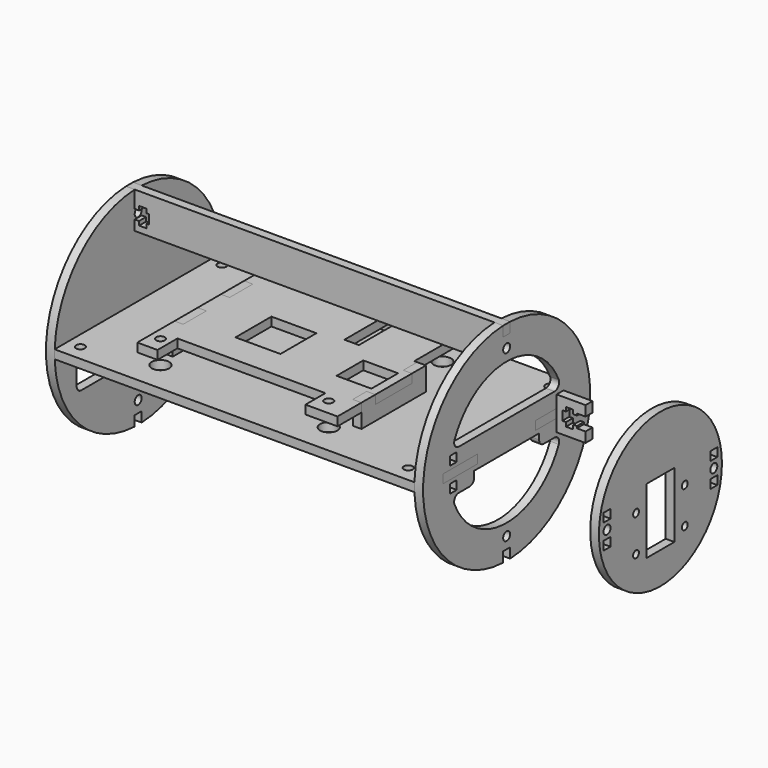
from build123d import *

# Parameters (mm, degrees)
F0_W      = 3
F0_H      = 15
F1_DEPTH  = 3
F3_R      = 1.5
F3_W      = 15.5
F3_H      = 15.5
F3_W_2    = 12
F3_H_2    = 11.5
F4_DEPTH  = 3
F5_W      = 3
F5_H      = 6
F5_W_2    = 10
F5_H_2    = 3
F5_W_3    = 7
F5_H_3    = 10
F6_DEPTH  = 25
F5_R      = 3
F5_R_2    = 1.5
F7_DEPTH  = 25
F9_DEPTH  = 3
F11_DEPTH = 3
F13_DEPTH = 3
F14_R     = 36
F14_W     = 25
F14_H     = 3
F15_DEPTH = 3
F16_R     = 2
F17_R     = 36
F17_W     = 15
F17_H     = 3
F18_DEPTH = 3
F19_R     = 1.5
F19_W     = 3
F19_H     = 7
F20_DEPTH = 130.001
F22_DEPTH = 3
F23_W     = 3
F23_H     = 3
F24_DEPTH = 3
F26_R     = 26.5
F26_W     = 3
F26_H     = 3
F26_R_2   = 1.25
F26_W_2   = 12
F26_H_2   = 22.5
F26_R_3   = 1.5
F27_DEPTH = 3
F28_R     = 1.524
F28_R_2   = 3
F29_DEPTH = 25


with BuildPart() as f1:
    # F0 (on Top) → F1 (new body)
    with BuildSketch(Plane.XY):
        Polygon((62, 36), (-62, 36), (-62, 27.5), (-62, 12.5), (-62, -12.5), (-62, -27.5), (-62, -36), (62, -36), (62, -27.5), (62, -12.5), (62, 12.5), (62, 27.5), align=None)
        with Locations((-63.5, 20)):
            Rectangle(F0_W, F0_H)
        with Locations((63.5, 20)):
            Rectangle(F0_W, F0_H)
        with Locations((-63.5, -20)):
            Rectangle(F0_W, F0_H)
        with Locations((63.5, -20)):
            Rectangle(F0_W, F0_H)
    extrude(amount=F1_DEPTH)


with BuildPart() as f4:
    # F3 (on offset) → F4 (new body)
    with BuildSketch(Plane(origin=(0, 0, 8), x_dir=(1, 0, 0), z_dir=(0, 0, -1))):
        Polygon((-37.5, 31), (-37.5, -31), (5, -31), (5, -5.1), (10, -5.1), (10, -31), (27.5, -31), (27.5, -7.1), (31.5, -7.1), (31.5, 31), (20.45, 31), (20.45, 22.4), (-30.55, 22.4), (-30.55, 31), align=None)
        with Locations((-34, -23.6)):
            Circle(F3_R, mode=Mode.SUBTRACT)
        with Locations((24, -23.6)):
            Circle(F3_R, mode=Mode.SUBTRACT)
        with Locations((-11, 4.4)):
            Rectangle(F3_W, F3_H, mode=Mode.SUBTRACT)
        with Locations((-34, 25.4)):
            Circle(F3_R, mode=Mode.SUBTRACT)
        with Locations((22.5, 6.9)):
            Rectangle(F3_W_2, F3_H_2, mode=Mode.SUBTRACT)
        with Locations((24, 25.4)):
            Circle(F3_R, mode=Mode.SUBTRACT)
    extrude(amount=-F4_DEPTH)


with BuildPart() as f6_tool:
    # F5 (on face) → F6 (new body)
    with BuildSketch(Plane.XY.offset(11)):
        with Locations((30, -17.68)):
            Rectangle(F5_W, F5_H)
        with Locations((30, 4.1)):
            Rectangle(F5_W, F5_H)
        with Locations((0, 29.5)):
            Rectangle(F5_W_2, F5_H_2)
        with Locations((-28, 29.5)):
            Rectangle(F5_W_3, F5_H_2)
        with Locations((-36, 10)):
            Rectangle(F5_W, F5_H_3)
        with Locations((-36, -10)):
            Rectangle(F5_W, F5_H_3)
    extrude(amount=-F6_DEPTH)


with BuildPart() as f1_1:
    add(f1.part)

    # F6: cut by f6_tool
    add(f6_tool.part, mode=Mode.SUBTRACT)

    # F5 (on face) → F7 (cut)
    with BuildSketch(Plane.XY.offset(11)):
        with Locations((24, -25.4)):
            Circle(F5_R)
        with Locations((24, -25.4)):
            Circle(F5_R_2, mode=Mode.SUBTRACT)
        with Locations((-34, -25.4)):
            Circle(F5_R)
        with Locations((-34, -25.4)):
            Circle(F5_R_2, mode=Mode.SUBTRACT)
        with Locations((24, 23.6)):
            Circle(F5_R)
        with Locations((24, 23.6)):
            Circle(F5_R_2, mode=Mode.SUBTRACT)
        with Locations((-34, 23.6)):
            Circle(F5_R)
        with Locations((-34, 23.6)):
            Circle(F5_R_2, mode=Mode.SUBTRACT)
    extrude(amount=-F7_DEPTH, mode=Mode.SUBTRACT)

    # F28 (on face) → F29 (cut)
    with BuildSketch(Plane(origin=(0, 0, 0), x_dir=(1, 0, 0), z_dir=(0, 0, -1))):
        with Locations((55.5, -30.5)):
            Circle(F28_R)
        with Locations((-57.5, -30.5)):
            Circle(F28_R)
        with Locations((-57.5, 30.5)):
            Circle(F28_R)
        with Locations((55.5, 30.5)):
            Circle(F28_R)
        with Locations((-34, 25.4)):
            Circle(F28_R_2)
        with Locations((24, 25.4)):
            Circle(F28_R_2)
        with Locations((-34, -23.6)):
            Circle(F28_R_2)
        with Locations((24, -23.6)):
            Circle(F28_R_2)
    extrude(amount=-F29_DEPTH, mode=Mode.SUBTRACT)


with BuildPart() as f4_1:
    add(f4.part)

    # F6: cut by f6_tool
    add(f6_tool.part, mode=Mode.SUBTRACT)


with BuildPart() as f9:
    # F8 (on face) → F9 (new body)
    with BuildSketch(Plane(origin=(-34.5, 0, 0), x_dir=(0, -1, 0), z_dir=(-1, 0, 0))):
        Polygon((5, 0), (15, 0), (15, 3), (19.5, 3), (19.5, 8), (15, 8), (15, 11), (5, 11), (5, 8), (-5, 8), (-5, 11), (-15, 11), (-15, 8), (-19.5, 8), (-19.5, 3), (-15, 3), (-15, 0), (-5, 0), (-5, 3), (5, 3), align=None)
    extrude(amount=F9_DEPTH)


with BuildPart() as f11:
    # F10 (on face) → F11 (new body)
    with BuildSketch(Plane(origin=(0, 28, 0), x_dir=(-1, 0, 0), z_dir=(0, 1, 0))):
        Polygon((5, 11), (-5, 11), (-5, 0), (5, 0), (5, 3), (24.5, 3), (24.5, 0), (31.5, 0), (31.5, 11), (24.5, 11), (24.5, 8), (5, 8), align=None)
    extrude(amount=F11_DEPTH)


with BuildPart() as f13:
    # F12 (on face) → F13 (new body)
    with BuildSketch(Plane.YZ.offset(28.5)):
        Polygon((7.1, 0), (7.1, 11), (1.1, 11), (1.1, 8), (-14.68, 8), (-14.68, 11), (-20.68, 11), (-20.68, 0), (-14.68, 0), (-14.68, 3), (1.1, 3), (1.1, 0), align=None)
    extrude(amount=F13_DEPTH)


with BuildPart() as f15:
    # F14 (on face) → F15 (new body)
    with BuildSketch(Plane.YZ.offset(62)):
        with Locations((0, 1.5)):
            Circle(F14_R)
        with BuildLine():
            ThreePointArc((-23.4787137637, 8.5), (0, 26), (23.4787137637, 8.5))
            ThreePointArc((23.4787137637, 8.5), (23.6554641744, 7.8772262541), (23.8156986041, 7.25))
            Line((23.8156986041, 7.25), (24.5, 7.25))
            Line((24.5, 7.25), (24.5, 4.25))
            Line((24.5, 4.25), (24.3451740598, 4.25))
            ThreePointArc((24.3451740598, 4.25), (24.4076097177, 3.625697031), (24.4540385213, 3))
            Line((24.4540385213, 3), (27.5, 3))
            Line((27.5, 3), (27.5, 0))
            Line((27.5, 0), (24.4540385213, 0))
            ThreePointArc((24.4540385213, 0), (24.4076097177, -0.625697031), (24.3451740598, -1.25))
            Line((24.3451740598, -1.25), (24.5, -1.25))
            Line((24.5, -1.25), (24.5, -4.25))
            Line((24.5, -4.25), (23.8156986041, -4.25))
            ThreePointArc((23.8156986041, -4.25), (23.6554641744, -4.8772262541), (23.4787137637, -5.5))
            ThreePointArc((23.4787137637, -5.5), (0, -23), (-23.4787137637, -5.5))
            ThreePointArc((-23.4787137637, -5.5), (-23.6554641744, -4.8772262541), (-23.8156986041, -4.25))
            Line((-23.8156986041, -4.25), (-24.5, -4.25))
            Line((-24.5, -4.25), (-24.5, -1.25))
            Line((-24.5, -1.25), (-24.3451740598, -1.25))
            ThreePointArc((-24.3451740598, -1.25), (-24.4076097177, -0.625697031), (-24.4540385213, 0))
            Line((-24.4540385213, 0), (-27.5, 0))
            Line((-27.5, 0), (-27.5, 3))
            Line((-27.5, 3), (-24.4540385213, 3))
            ThreePointArc((-24.4540385213, 3), (-24.4076097177, 3.625697031), (-24.3451740598, 4.25))
            Line((-24.3451740598, 4.25), (-24.5, 4.25))
            Line((-24.5, 4.25), (-24.5, 7.25))
            Line((-24.5, 7.25), (-23.8156986041, 7.25))
            ThreePointArc((-23.8156986041, 7.25), (-23.6554641744, 7.8772262541), (-23.4787137637, 8.5))
        make_face(mode=Mode.SUBTRACT)
        with BuildLine():
            Line((-12.5, 0), (-24.4540385213, 0))
            ThreePointArc((-24.4540385213, 0), (-24.4076097177, -0.625697031), (-24.3451740598, -1.25))
            Line((-24.3451740598, -1.25), (-21.5, -1.25))
            Line((-21.5, -1.25), (-21.5, -4.25))
            Line((-21.5, -4.25), (-23.8156986041, -4.25))
            ThreePointArc((-23.8156986041, -4.25), (-23.6554641744, -4.8772262541), (-23.4787137637, -5.5))
            Line((-23.4787137637, -5.5), (-14, -5.5))
            Line((-14, -5.5), (-14, -1.5))
            Line((-14, -1.5), (14, -1.5))
            Line((14, -1.5), (14, -5.5))
            Line((14, -5.5), (23.4787137637, -5.5))
            ThreePointArc((23.4787137637, -5.5), (23.6554641744, -4.8772262541), (23.8156986041, -4.25))
            Line((23.8156986041, -4.25), (21.5, -4.25))
            Line((21.5, -4.25), (21.5, -1.25))
            Line((21.5, -1.25), (24.3451740598, -1.25))
            ThreePointArc((24.3451740598, -1.25), (24.4076097177, -0.625697031), (24.4540385213, 0))
            Line((24.4540385213, 0), (12.5, 0))
            Line((12.5, 0), (-12.5, 0))
        make_face()
        with BuildLine():
            ThreePointArc((23.8156986041, 7.25), (23.6554641744, 7.8772262541), (23.4787137637, 8.5))
            Line((23.4787137637, 8.5), (-23.4787137637, 8.5))
            ThreePointArc((-23.4787137637, 8.5), (-23.6554641744, 7.8772262541), (-23.8156986041, 7.25))
            Line((-23.8156986041, 7.25), (-21.5, 7.25))
            Line((-21.5, 7.25), (-21.5, 4.25))
            Line((-21.5, 4.25), (-24.3451740598, 4.25))
            ThreePointArc((-24.3451740598, 4.25), (-24.4076097177, 3.625697031), (-24.4540385213, 3))
            Line((-24.4540385213, 3), (-12.5, 3))
            Line((-12.5, 3), (12.5, 3))
            Line((12.5, 3), (24.4540385213, 3))
            ThreePointArc((24.4540385213, 3), (24.4076097177, 3.625697031), (24.3451740598, 4.25))
            Line((24.3451740598, 4.25), (21.5, 4.25))
            Line((21.5, 4.25), (21.5, 7.25))
            Line((21.5, 7.25), (23.8156986041, 7.25))
        make_face()
        with Locations((0, 1.5)):
            Rectangle(F14_W, F14_H)
    extrude(amount=F15_DEPTH)

    # F16
    f16_edges = [f15.edges().sort_by_distance(p)[0] for p in [
        (63.5, 14, -5.5),
        (63.5, -14, -5.5),
        (63.5, 23.478714, -5.5),
        (63.5, 23.478714, 8.5),
        (63.5, -23.478714, 8.5),
        (63.5, -23.478714, -5.5),
    ]]
    fillet(f16_edges, radius=F16_R)


with BuildPart() as f18:
    # F17 (on face) → F18 (new body)
    with BuildSketch(Plane(origin=(-62, 0, 0), x_dir=(0, -1, 0), z_dir=(-1, 0, 0))):
        with Locations((0, 1.5)):
            Circle(F17_R)
        with BuildLine():
            ThreePointArc((26.5, -12.1), (25.9142135624, -13.5142135624), (24.5, -14.1))
            Line((24.5, -14.1), (-24.5, -14.1))
            ThreePointArc((-24.5, -14.1), (-25.9142135624, -13.5142135624), (-26.5, -12.1))
            Line((-26.5, -12.1), (-26.5, -4))
            ThreePointArc((-26.5, -4), (-25.9142135624, -2.5857864376), (-24.5, -2))
            Line((-24.5, -2), (24.5, -2))
            ThreePointArc((24.5, -2), (25.9142135624, -2.5857864376), (26.5, -4))
            Line((26.5, -4), (26.5, -12.1))
        make_face(mode=Mode.SUBTRACT)
        with Locations((-20, 1.5)):
            Rectangle(F17_W, F17_H, mode=Mode.SUBTRACT)
        with Locations((20, 1.5)):
            Rectangle(F17_W, F17_H, mode=Mode.SUBTRACT)
    extrude(amount=F18_DEPTH)


with BuildPart() as f20_tool:
    # F19 (on face) → F20 (new body, through all)
    with BuildSketch(Plane.YZ.offset(65)):
        with Locations((0, -27)):
            Circle(F19_R)
        with Locations((0, 30)):
            Circle(F19_R)
        with Locations((0, -34.5)):
            Rectangle(F19_W, F19_H)
        with Locations((0, 37.5)):
            Rectangle(F19_W, F19_H)
    extrude(amount=-F20_DEPTH)


with BuildPart() as f15_1:
    add(f15.part)

    # F20: cut by f20_tool
    add(f20_tool.part, mode=Mode.SUBTRACT)


with BuildPart() as f18_1:
    add(f18.part)

    # F20: cut by f20_tool
    add(f20_tool.part, mode=Mode.SUBTRACT)


with BuildPart() as f22:
    # F21 (on face) → F22 (new body)
    with BuildSketch(Plane(origin=(0, -1.5, 0), x_dir=(-1, 0, 0), z_dir=(0, 1, 0))):
        Polygon((-65, 37.4687364248), (-65, 34), (-62, 34), (-62, 31.6), (-60.5, 31.6), (-60.5, 33), (-58, 33), (-58, 31.6), (-57, 31.6), (-57, 28.4), (-58, 28.4), (-58, 27), (-60.5, 27), (-60.5, 28.4), (-62, 28.4), (-62, 24.9), (62, 24.9), (62, 28.4), (60.5, 28.4), (60.5, 27), (58, 27), (58, 28.4), (57, 28.4), (57, 31.6), (58, 31.6), (58, 33), (60.5, 33), (60.5, 31.6), (62, 31.6), (62, 34), (65, 34), (65, 37.4687364248), align=None)
    extrude(amount=F22_DEPTH)


with BuildPart() as f24:
    # F23 (on face) → F24 (new body)
    with BuildSketch(Plane.XZ.offset(-24.5)):
        Polygon((65, -1.25), (65, -4.25), (75, -4.25), (75, -0.75), (72, -0.75), (72, -0.1), (70.75, -0.1), (70.75, -1.5), (68.25, -1.5), (68.25, -0.1), (67, -0.1), (67, 3.1), (68.25, 3.1), (68.25, 4.5), (70.75, 4.5), (70.75, 3.1), (72, 3.1), (72, 3.75), (75, 3.75), (75, 7.25), (65, 7.25), (62, 7.25), (62, 4.25), (65, 4.25), align=None)
        with Locations((63.5, -2.75)):
            Rectangle(F23_W, F23_H)
    extrude(amount=F24_DEPTH)


with BuildPart() as f27:
    # F26 (on offset) → F27 (new body)
    with BuildSketch(Plane.YZ.offset(115)):
        with Locations((0, 1.5)):
            Circle(F26_R)
        with Locations((-23, -2.75)):
            Rectangle(F26_W, F26_H, mode=Mode.SUBTRACT)
        with Locations((-10.5, -11)):
            Circle(F26_R_2, mode=Mode.SUBTRACT)
        with Locations((10.5, -11)):
            Circle(F26_R_2, mode=Mode.SUBTRACT)
        with Locations((0, -2.75)):
            Rectangle(F26_W_2, F26_H_2, mode=Mode.SUBTRACT)
        with Locations((23, -2.75)):
            Rectangle(F26_W, F26_H, mode=Mode.SUBTRACT)
        with Locations((-23, 1.5)):
            Circle(F26_R_3, mode=Mode.SUBTRACT)
        with Locations((-23, 5.75)):
            Rectangle(F26_W, F26_H, mode=Mode.SUBTRACT)
        with Locations((-10.5, 1.5)):
            Circle(F26_R_2, mode=Mode.SUBTRACT)
        with Locations((10.5, 1.5)):
            Circle(F26_R_2, mode=Mode.SUBTRACT)
        with Locations((23, 1.5)):
            Circle(F26_R_3, mode=Mode.SUBTRACT)
        with Locations((23, 5.75)):
            Rectangle(F26_W, F26_H, mode=Mode.SUBTRACT)
    extrude(amount=F27_DEPTH)


solid = Compound([f1_1.part, f4_1.part, f9.part, f11.part, f13.part, f15_1.part, f18_1.part, f22.part, f24.part, f27.part])
